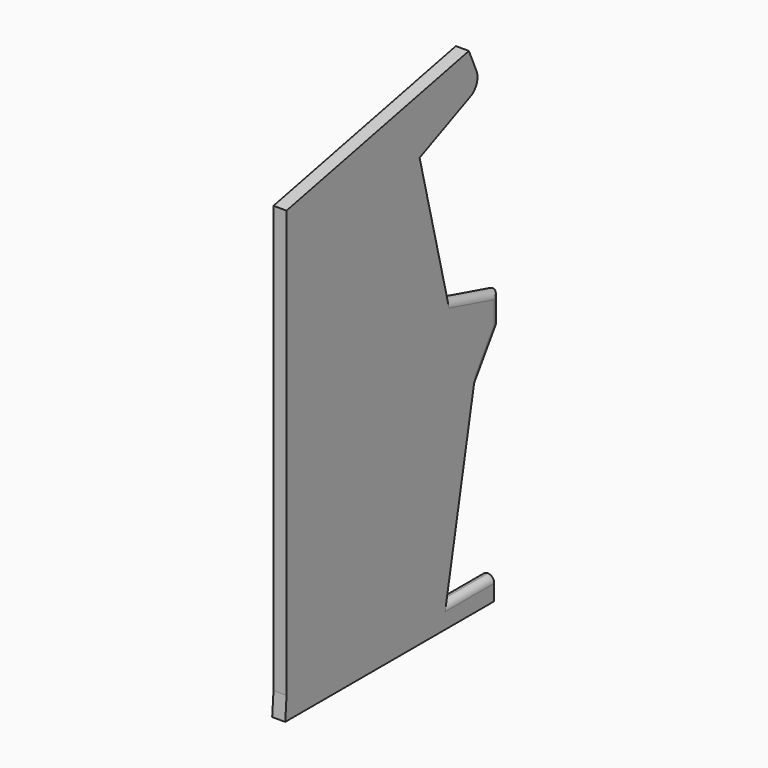
from build123d import *

# Parameters (mm, degrees)
F1_DEPTH     = 3.81
F2_R         = 2.032
F3_T1_DEPTH  = 18.831700203
F3_T6_DEPTH  = 29.7046687957
F3_T11_DEPTH = 27.9890917976
F4_R         = 4.2926
F5_R         = 2.032
F6_T4_DEPTH  = 27.583079529


# Not quite as in the source:
# - a fillet or chamfer that OpenCascade refuses, or shapes differently, is made with other operations: its cross-section is extruded or revolved along the edge and cut away or added


with BuildPart() as f1:
    # F0 (on Right) → F1 (new body)
    with BuildSketch(Plane.YZ):
        Polygon((-45.0965359712, 64.4910041714), (-45.0965359712, 37.5272747601), (-45.0965359712, 31.8507016177), (-45.0965359712, -59.9205825006), (-45.5695882344, -66.5432545816), (30.5911183453, -66.5432545816), (30.5911183453, -59.9205825006), (13.0883513114, -59.9205825006), (22.5493062383, -11.1966548016), (32.4833087719, 3.7043508614), (32.4833087719, 12.4557385693), (13.561398918, 17.6592650363), (3.3908628023, 58.3413843537), (25.8606404162, 68.2753812993), (21.3563181986, 78.4637394279), align=None)
    extrude(amount=-F1_DEPTH)

    # F2
    f2_edges = [f1.edges().sort_by_distance(p)[0] for p in [
        (0, 23.022354, 15.057502),
        (0, 27.516308, -3.746152),
        (0, 32.483309, 8.080045),
    ]]
    fillet(f2_edges, radius=F2_R)

    # F3: fillet of radius 2.032 on 3 edges, made by hand

    # F3_s2 → F3_t1 (cut)
    with BuildSketch(Plane.XY.offset(-1.3358053862)):
        with BuildLine():
            ThreePointArc((-3.81, 30.4672462728), (-3.302, 31.8112879389), (-2.032, 32.4833087719))
            Line((-2.032, 32.4833087719), (-2.03708, 32.5236300218))
            ThreePointArc((-2.03708, 32.5236300218), (-2.921, 32.5239487719), (-3.81, 32.5239487719))
            Line((-3.81, 32.5239487719), (-3.85064, 32.4833087719))
            Line((-3.85064, 32.4833087719), (-3.85064, 30.4672462728))
            Line((-3.85064, 30.4672462728), (-3.81, 30.4672462728))
        make_face()
    extrude(amount=F3_T1_DEPTH, mode=Mode.SUBTRACT)


with BuildPart() as f3_tool4:
    # F3_s5 → F3_t6 (new body)
    with BuildSketch(Plane(origin=(0, 31.8747173735, -8.7655493956), x_dir=(1, 0, 0), z_dir=(0, -0.9642053764, 0.2651565426))):
        with BuildLine():
            ThreePointArc((-2.032, 20.6230519415), (-3.302, 19.9510311084), (-3.81, 18.6069894424))
            Line((-3.81, 18.6069894424), (-3.85064, 18.6069894424))
            Line((-3.85064, 18.6069894424), (-3.85064, 20.6230519415))
            Line((-3.85064, 20.6230519415), (-3.81, 20.6636919415))
            ThreePointArc((-3.81, 20.6636919415), (-2.921, 20.6636919415), (-2.03708, 20.6633731914))
            Line((-2.03708, 20.6633731914), (-2.032, 20.6230519415))
        make_face()
    extrude(amount=F3_T6_DEPTH)

    split(bisect_by=Plane(origin=(0, 16.9187920929, 4.2297006376), x_dir=(1, 0, 0), z_dir=(0, 0.9701424649, 0.2425357661)), keep=Keep.TOP)


with BuildPart() as f1_1:
    add(f1.part)

    # F3_t3: cut F3_tool4
    add(f3_tool4.part, mode=Mode.SUBTRACT)


with BuildPart() as f3_tool9:
    # F3_s10 → F3_t11 (new body)
    with BuildSketch(Plane(origin=(0, -1.0252151282, -1.5378228845), x_dir=(1, 0, 0), z_dir=(0, 0.5547001482, 0.8320503263))):
        with BuildLine():
            ThreePointArc((-3.81, 22.9568811933), (-3.302, 24.3009228594), (-2.032, 24.9729436924))
            Line((-2.032, 24.9729436924), (-2.03708, 25.0132649423))
            ThreePointArc((-2.03708, 25.0132649423), (-2.921, 25.0135836924), (-3.81, 25.0135836924))
            Line((-3.81, 25.0135836924), (-3.85064, 24.9729436924))
            Line((-3.85064, 24.9729436924), (-3.85064, 22.9568811933))
            Line((-3.85064, 22.9568811933), (-3.81, 22.9568811933))
        make_face()
    extrude(amount=F3_T11_DEPTH)

    split(bisect_by=Plane(origin=(0, 23.8251156296, -4.6262351117), x_dir=(1, 0, 0), z_dir=(0, 0.981664966, -0.1906145181)), keep=Keep.TOP)


with BuildPart() as f1_2:
    add(f1_1.part)

    # F3_t8: cut F3_tool9
    add(f3_tool9.part, mode=Mode.SUBTRACT)

    # F4
    f4_edges = [f1_2.edges().sort_by_distance(p)[0] for p in [
        (-1.905, 25.86064, 68.275381),
    ]]
    fillet(f4_edges, radius=F4_R)

    # F5
    f5_edges = [f1_2.edges().sort_by_distance(p)[0] for p in [
        (-3.81, 21.839735, -59.920583),
    ]]
    fillet(f5_edges, radius=F5_R)

    # F6: fillet of radius 2.032 on 1 edges, made by hand


with BuildPart() as f6_tool2:
    # F6_s3 → F6_t4 (new body)
    with BuildSketch(Plane.XZ.offset(-35.6312745929)):
        with BuildLine():
            ThreePointArc((-1.778, -59.9205825006), (-0.508, -60.5926033336), (0, -61.9366449997))
            Line((0, -61.9366449997), (0, -59.9205825006))
            Line((0, -59.9205825006), (-1.778, -59.9205825006))
        make_face()
    extrude(amount=F6_T4_DEPTH)

    split(bisect_by=Plane(origin=(0, 23.8251156296, -4.6262351117), x_dir=(1, 0, 0), z_dir=(0, 0.981664966, -0.1906145181)), keep=Keep.TOP)


with BuildPart() as f1_3:
    add(f1_2.part)

    # F6_t1: cut F6_tool2
    add(f6_tool2.part, mode=Mode.SUBTRACT)


solid = f1_3.part
